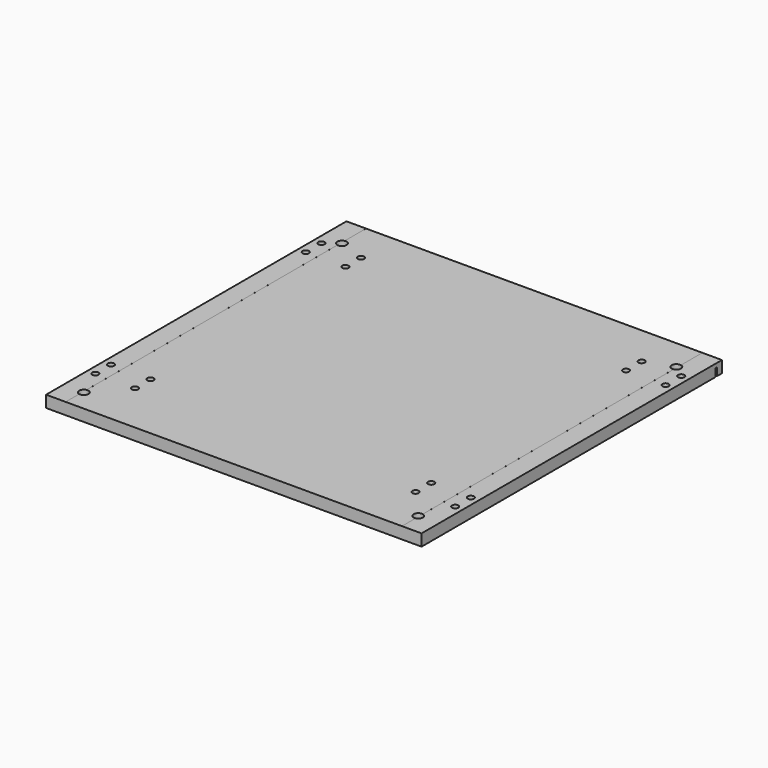
from build123d import *

# Parameters (mm, degrees)
F0_W      = 609.6
F0_H      = 609.6
F0_R      = 7.540625
F0_R_2    = 5.159375
F1_DEPTH  = 19.05
F2_DEPTH  = 12.7
F3_W      = 609.6
F3_H      = 3.175
F4_DEPTH  = 12.7
F5_R      = 9.525
F6_DEPTH  = 6.35
F7_W      = 25.4
F7_H      = 0.0254
F7_W_2    = 50
F8_DEPTH  = 0.254
F10_DEPTH = 2.54


# Not quite as in the source:
# - a pattern or mirror of a feature is missing from the dataset's text; its kind, count and spacing are read off the source's solid


with BuildPart() as f1:
    # F0 (on Top) → F1 (new body)
    with BuildSketch(Plane.XY):
        Rectangle(F0_W, F0_H)
        with Locations((-271.4625, -269.875)):
            Circle(F0_R, mode=Mode.SUBTRACT)
        with Locations((-292.1, -220.6625)):
            Circle(F0_R_2, mode=Mode.SUBTRACT)
        with Locations((-292.1, -188.9125)):
            Circle(F0_R_2, mode=Mode.SUBTRACT)
        with Locations((-227.80625, -220.6625)):
            Circle(F0_R_2, mode=Mode.SUBTRACT)
        with Locations((-227.80625, -188.9125)):
            Circle(F0_R_2, mode=Mode.SUBTRACT)
        with Locations((-292.1, 206.375)):
            Circle(F0_R_2, mode=Mode.SUBTRACT)
        with Locations((-227.80625, 206.375)):
            Circle(F0_R_2, mode=Mode.SUBTRACT)
        with Locations((-292.1, 238.125)):
            Circle(F0_R_2, mode=Mode.SUBTRACT)
        with Locations((-271.4625, 254)):
            Circle(F0_R, mode=Mode.SUBTRACT)
        with Locations((-227.80625, 238.125)):
            Circle(F0_R_2, mode=Mode.SUBTRACT)
        with Locations((-271.4625, 254)):
            Circle(F0_R)
        with Locations((-292.1, 238.125)):
            Circle(F0_R_2)
        with Locations((-292.1, 206.375)):
            Circle(F0_R_2)
        with Locations((-227.80625, 206.375)):
            Circle(F0_R_2)
        with Locations((-227.80625, 238.125)):
            Circle(F0_R_2)
        with Locations((-227.80625, -188.9125)):
            Circle(F0_R_2)
        with Locations((-227.80625, -220.6625)):
            Circle(F0_R_2)
        with Locations((-292.1, -220.6625)):
            Circle(F0_R_2)
        with Locations((-292.1, -188.9125)):
            Circle(F0_R_2)
        with Locations((-271.4625, -269.875)):
            Circle(F0_R)
    extrude(amount=-F1_DEPTH)

    # F0 (on Top) → F2 (cut)
    with BuildSketch(Plane.XY):
        with Locations((-271.4625, -269.875)):
            Circle(F0_R)
        with Locations((-292.1, -220.6625)):
            Circle(F0_R_2)
        with Locations((-227.80625, -220.6625)):
            Circle(F0_R_2)
        with Locations((-227.80625, -188.9125)):
            Circle(F0_R_2)
        with Locations((-292.1, -188.9125)):
            Circle(F0_R_2)
        with Locations((-292.1, 206.375)):
            Circle(F0_R_2)
        with Locations((-227.80625, 206.375)):
            Circle(F0_R_2)
        with Locations((-227.80625, 238.125)):
            Circle(F0_R_2)
        with Locations((-292.1, 238.125)):
            Circle(F0_R_2)
        with Locations((-271.4625, 254)):
            Circle(F0_R)
    f2 = extrude(amount=-F2_DEPTH, mode=Mode.SUBTRACT)

    # F2_copies: F2 across plane
    add(f2.mirror(Plane(origin=(0, 0, 0), x_dir=(0, 0, 1), z_dir=(1, 0, 0))), mode=Mode.SUBTRACT)

    # F3 (on face) → F4 (cut)
    with BuildSketch(Plane(origin=(0, 0, -19.05), x_dir=(1, 0, 0), z_dir=(0, 0, -1))):
        with Locations((0, -293.6875)):
            Rectangle(F3_W, F3_H)
    extrude(amount=-F4_DEPTH, mode=Mode.SUBTRACT)

    # F5 (on face) → F6 (cut)
    with BuildSketch(Plane(origin=(0, 0, -19.05), x_dir=(1, 0, 0), z_dir=(0, 0, -1))):
        with Locations((260.35, -274.6375)):
            Circle(F5_R)
        with Locations((204.7875, -274.6375)):
            Circle(F5_R)
        with Locations((204.7875, -232.56875)):
            Circle(F5_R)
        with Locations((260.35, -232.56875)):
            Circle(F5_R)
        with Locations((-204.7875, -274.6375)):
            Circle(F5_R)
        with Locations((-260.35, -274.6375)):
            Circle(F5_R)
        with Locations((-260.35, -232.56875)):
            Circle(F5_R)
        with Locations((-204.7875, -232.56875)):
            Circle(F5_R)
        with Locations((-204.7875, 205.58125)):
            Circle(F5_R)
        with Locations((-260.35, 205.58125)):
            Circle(F5_R)
        with Locations((-260.35, 247.65)):
            Circle(F5_R)
        with Locations((-204.7875, 247.65)):
            Circle(F5_R)
        with Locations((204.7875, 247.65)):
            Circle(F5_R)
        with Locations((204.7875, 205.58125)):
            Circle(F5_R)
        with Locations((260.35, 205.58125)):
            Circle(F5_R)
        with Locations((260.35, 247.65)):
            Circle(F5_R)
    extrude(amount=-F6_DEPTH, mode=Mode.SUBTRACT)

    # F7 (on face) → F8 (cut)
    with BuildSketch(Plane(origin=(0, 0, -19.05), x_dir=(1, 0, 0), z_dir=(0, 0, -1))):
        with Locations((-156.0546457767, -265.0721735465)):
            Rectangle(F7_W, F7_H)
        with Locations((-145.1898425817, -234.882380328)):
            Rectangle(F7_W_2, F7_H)
    extrude(amount=-F8_DEPTH, mode=Mode.SUBTRACT)

    # F9 (on face) → F10 (cut)
    with BuildSketch(Plane.XY):
        with BuildLine():
            Line((-273.0246, 304.8), (-273.05, 304.8))
            Line((-273.05, 304.8), (-273.05, 261.3716259496))
            ThreePointArc((-273.05, 261.3716259496), (-273.0373023354, 261.3743489879), (-273.0246, 261.3770501544))
            Line((-273.0246, 261.3770501544), (-273.0246, 304.8))
        make_face()
        with BuildLine():
            ThreePointArc((-273.0246, 261.3770501544), (-273.0373023354, 261.3743489879), (-273.05, 261.3716259496))
            Line((-273.05, 261.3716259496), (-273.05, 246.6283740504))
            ThreePointArc((-273.05, 246.6283740504), (-273.0373023354, 246.6256510121), (-273.0246, 246.6229498456))
            Line((-273.0246, 246.6229498456), (-273.0246, 261.3770501544))
        make_face()
        with BuildLine():
            Line((273.05, 304.8), (273.0246, 304.8))
            Line((273.0246, 304.8), (273.0246, 261.3770501544))
            ThreePointArc((273.0246, 261.3770501544), (273.0373023354, 261.3743489879), (273.05, 261.3716259496))
            Line((273.05, 261.3716259496), (273.05, 304.8))
        make_face()
        with BuildLine():
            ThreePointArc((-273.0246, 246.6229498456), (-273.0373023354, 246.6256510121), (-273.05, 246.6283740504))
            Line((-273.05, 246.6283740504), (-273.05, -262.5033740504))
            ThreePointArc((-273.05, -262.5033740504), (-273.0373023354, -262.5006510121), (-273.0246, -262.4979498456))
            Line((-273.0246, -262.4979498456), (-273.0246, 246.6229498456))
        make_face()
        with BuildLine():
            ThreePointArc((-273.0246, -262.4979498456), (-273.0373023354, -262.5006510121), (-273.05, -262.5033740504))
            Line((-273.05, -262.5033740504), (-273.05, -277.2466259496))
            ThreePointArc((-273.05, -277.2466259496), (-273.0373023354, -277.2493489879), (-273.0246, -277.2520501544))
            Line((-273.0246, -277.2520501544), (-273.0246, -262.4979498456))
        make_face()
        with BuildLine():
            Line((-273.05, -277.2466259496), (-273.05, -304.8))
            Line((-273.05, -304.8), (-273.0246, -304.8))
            Line((-273.0246, -304.8), (-273.0246, -277.2520501544))
            ThreePointArc((-273.0246, -277.2520501544), (-273.0373023354, -277.2493489879), (-273.05, -277.2466259496))
        make_face()
        with BuildLine():
            ThreePointArc((273.05, 246.6283740504), (273.0373023354, 246.6256510121), (273.0246, 246.6229498456))
            Line((273.0246, 246.6229498456), (273.0246, -262.4979498456))
            ThreePointArc((273.0246, -262.4979498456), (273.0373023354, -262.5006510121), (273.05, -262.5033740504))
            Line((273.05, -262.5033740504), (273.05, 246.6283740504))
        make_face()
        with BuildLine():
            Line((273.0246, -277.2520501544), (273.0246, -304.8))
            Line((273.0246, -304.8), (273.05, -304.8))
            Line((273.05, -304.8), (273.05, -277.2466259496))
            ThreePointArc((273.05, -277.2466259496), (273.0373023354, -277.2493489879), (273.0246, -277.2520501544))
        make_face()
    extrude(amount=-F10_DEPTH, mode=Mode.SUBTRACT)


solid = f1.part
